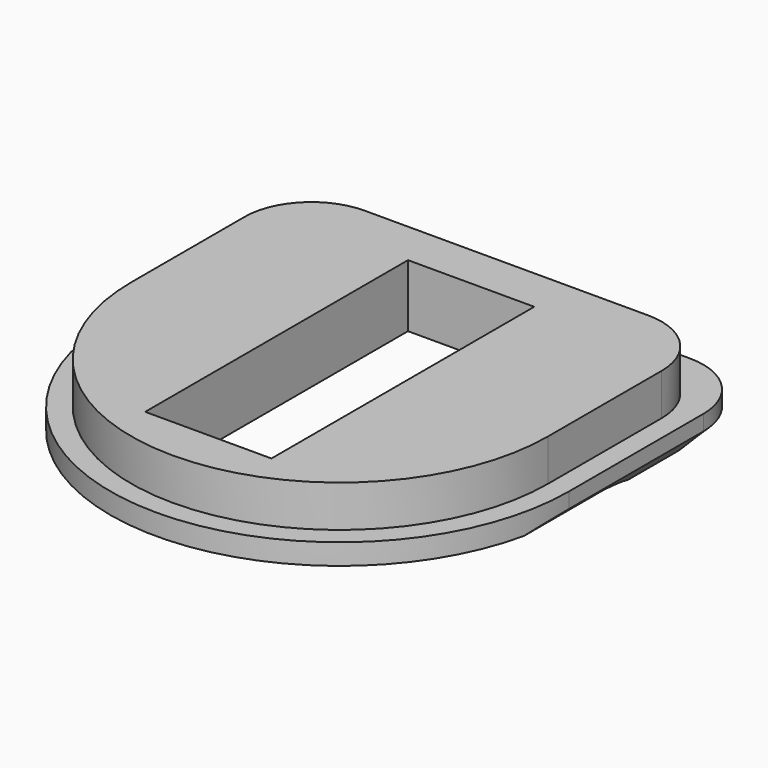
from build123d import *

# Parameters (mm, degrees)
F1_DEPTH    = 3.175
F3_DEPTH    = 3.175
F5_DEPTH    = 1.5875
F6_W        = 9.6138492227
F6_H        = 25.0137764961
F7_DEPTH    = 25.4
F8_R        = 5.08
F9_T1_DEPTH = 21.5230971591
F9_T3_DEPTH = 24.765
F9_T6_ANGLE = 90
F9_T8_ANGLE = 90


# Not quite as in the source:
# - a fillet or chamfer that OpenCascade refuses, or shapes differently, is made with other operations: its cross-section is extruded or revolved along the edge and cut away or added


with BuildPart() as f1:
    # F0 (on Top) → F1 (new body)
    with BuildSketch(Plane.XY):
        with BuildLine():
            ThreePointArc((-17.4625, 0), (0, -17.4625), (17.4625, 0))
            ThreePointArc((17.4625, 0), (0, 17.4625), (-17.4625, 0))
        make_face()
        with BuildLine():
            ThreePointArc((-17.4625, 0), (0, 17.4625), (17.4625, 0))
            Line((17.4625, 0), (17.4625, 17.859375))
            Line((17.4625, 17.859375), (-17.4625, 17.859375))
            Line((-17.4625, 17.859375), (-17.4625, 0))
        make_face()
    extrude(amount=F1_DEPTH)

    # F2 (on face) → F3 (join)
    with BuildSketch(Plane.XY.offset(3.175)):
        with BuildLine():
            ThreePointArc((-5.44e-08, 15.875), (-11.2253201706, 11.2253201321), (-15.875, 0))
            ThreePointArc((-15.875, 0), (0, -15.875), (15.875, 0))
            ThreePointArc((15.875, 0), (11.2253201321, 11.2253201706), (-5.44e-08, 15.875))
        make_face()
        with BuildLine():
            Line((-15.875, 15.875), (-15.875, 0))
            ThreePointArc((-15.875, 0), (-11.2253201706, 11.2253201321), (-5.44e-08, 15.875))
            Line((-5.44e-08, 15.875), (-15.875, 15.875))
        make_face()
        with BuildLine():
            ThreePointArc((-5.44e-08, 15.875), (11.2253201321, 11.2253201706), (15.875, 0))
            Line((15.875, 0), (15.875, 15.875))
            Line((15.875, 15.875), (-5.44e-08, 15.875))
        make_face()
    extrude(amount=F3_DEPTH)

    # F4 (on face) → F5 (cut)
    with BuildSketch(Plane(origin=(0, 0, 0), x_dir=(1, 0, 0), z_dir=(0, 0, -1))):
        with BuildLine():
            ThreePointArc((-17.4625, 0), (0, -17.4625), (17.4625, 0))
            ThreePointArc((17.4625, 0), (0, 17.4625), (-17.4625, 0))
        make_face()
    extrude(amount=-F5_DEPTH, mode=Mode.SUBTRACT)

    # F6 (on face) → F7 (cut)
    with BuildSketch(Plane(origin=(0, 0, 1.5875), x_dir=(1, 0, 0), z_dir=(0, 0, -1))):
        Rectangle(F6_W, F6_H)
    extrude(amount=-F7_DEPTH, mode=Mode.SUBTRACT)

    # F8
    f8_edges = [f1.edges().sort_by_distance(p)[0] for p in [
        (17.4625, 17.859375, 1.5875),
        (-17.4625, 17.859375, 1.5875),
        (-15.875, 15.875, 4.7625),
        (15.875, 15.875, 4.7625),
    ]]
    fillet(f8_edges, radius=F8_R)

    # F9: chamfer of 2 on 2 edges, made by hand

    # F9_s2 → F9_t1 (cut)
    with BuildSketch(Plane.XZ.offset(-12.779375)):
        Polygon((17.4625, 2), (15.4625, 0), (17.4625, 0), align=None)
        Polygon((-15.4625, 0), (-17.4625, 2), (-17.4625, 0), align=None)
    extrude(amount=F9_T1_DEPTH, mode=Mode.SUBTRACT)

    # F9_s4 → F9_t3 (cut)
    with BuildSketch(Plane.YZ.offset(-12.3825)):
        Polygon((15.859375, 0), (17.859375, 2), (17.859375, 0), align=None)
    extrude(amount=F9_T3_DEPTH, mode=Mode.SUBTRACT)

    # F9_s5 → F9_t6 (revolve, cut)
    with BuildSketch(Plane.XZ.offset(-12.779375)):
        Polygon((15.4625, 0), (17.4625, 2), (17.4625, 0), align=None)
    revolve(axis=Axis((12.3825, 12.779375, 0), (0, 0, 1)), revolution_arc=F9_T6_ANGLE, mode=Mode.SUBTRACT)

    # F9_s7 → F9_t8 (revolve, cut)
    with BuildSketch(Plane.YZ.offset(-12.3825)):
        Polygon((15.859375, 0), (17.859375, 2), (17.859375, 0), align=None)
    revolve(axis=Axis((-12.3825, 12.779375, 0), (0, 0, 1)), revolution_arc=F9_T8_ANGLE, mode=Mode.SUBTRACT)


solid = f1.part
